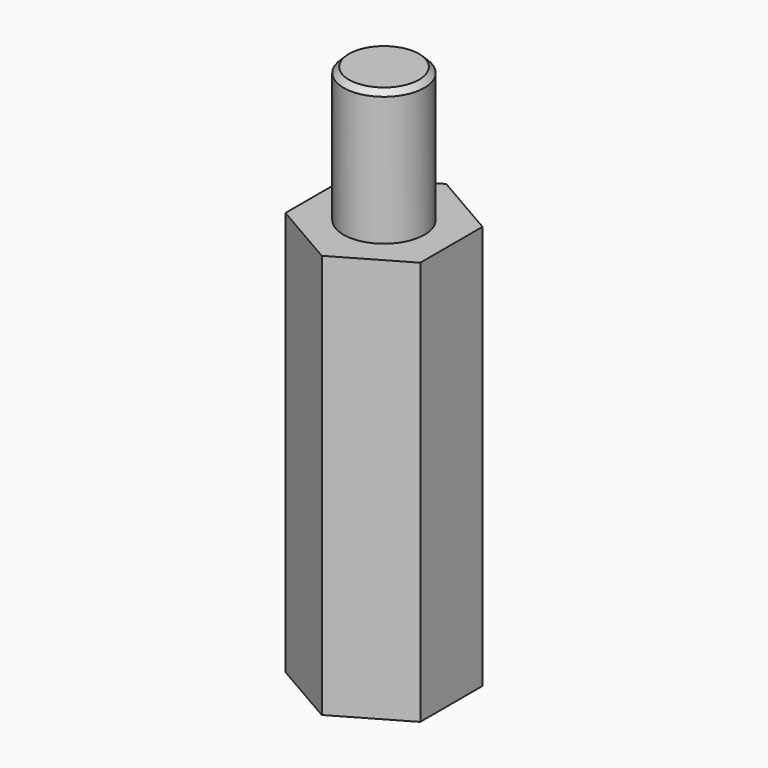
from build123d import *

# Parameters (mm, degrees)
F0_R     = 1.5
F1_DEPTH = 15
F2_DEPTH = 20
F3_SIZE  = 0.2
F4_DEPTH = 2.5


# Not quite as in the source:
# - a feature names something its author has since deleted; it is built from what else it names


with BuildPart() as f1:
    # F0 (on Top) → F1 (new body)
    with BuildSketch(Plane.XY):
        Polygon((-6.5392298422, -1.443375673), (-6.5392298422, 1.443375673), (-9.0392298422, 2.8867513459), (-11.5392298422, 1.443375673), (-11.5392298422, -1.443375673), (-9.0392298422, -2.8867513459), align=None)
        with Locations((-9.0392298422, 0)):
            Circle(F0_R, mode=Mode.SUBTRACT)
    extrude(amount=F1_DEPTH)

    # F0 (on Top) → F2 (join)
    with BuildSketch(Plane.XY):
        with Locations((-9.0392298422, 0)):
            Circle(F0_R)
    extrude(amount=F2_DEPTH)

    # F3
    f3_edges = [f1.edges().sort_by_distance(p)[0] for p in [
        (-10.53923, 0, 20),
    ]]
    chamfer(f3_edges, length=F3_SIZE)

    # F0 (on Top) → F4 (cut)
    with BuildSketch(Plane.XY):
        with Locations((-9.0392298422, 0)):
            Circle(F0_R)
    extrude(amount=F4_DEPTH, mode=Mode.SUBTRACT)


solid = f1.part
